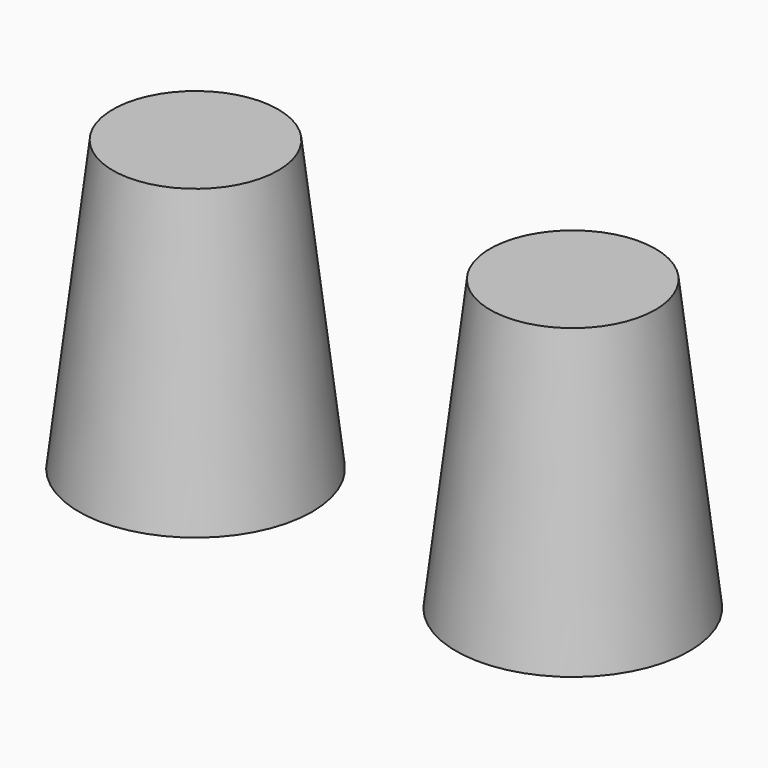
from build123d import *

# Parameters (mm, degrees)
F0_R     = 25
F1_DEPTH = 62
F1_TAPER = 6.7


# Not quite as in the source:
# - a feature of the source that left no trace in its solid (it failed there, or was rolled back) is left out


with BuildPart() as f1:
    # F0 (on Top) → F1 (new body)
    with BuildSketch(Plane.XY):
        with Locations((-43.0139228702, 0)):
            Circle(F0_R)
    extrude(amount=F1_DEPTH, taper=F1_TAPER)


with BuildPart() as f1b:
    # F0 (on Top) → F1, piece 2 (new body)
    with BuildSketch(Plane.XY):
        with Locations((37.7888046205, 0)):
            Circle(F0_R)
    extrude(amount=F1_DEPTH, taper=F1_TAPER)


solid = Compound([f1.part, f1b.part])
